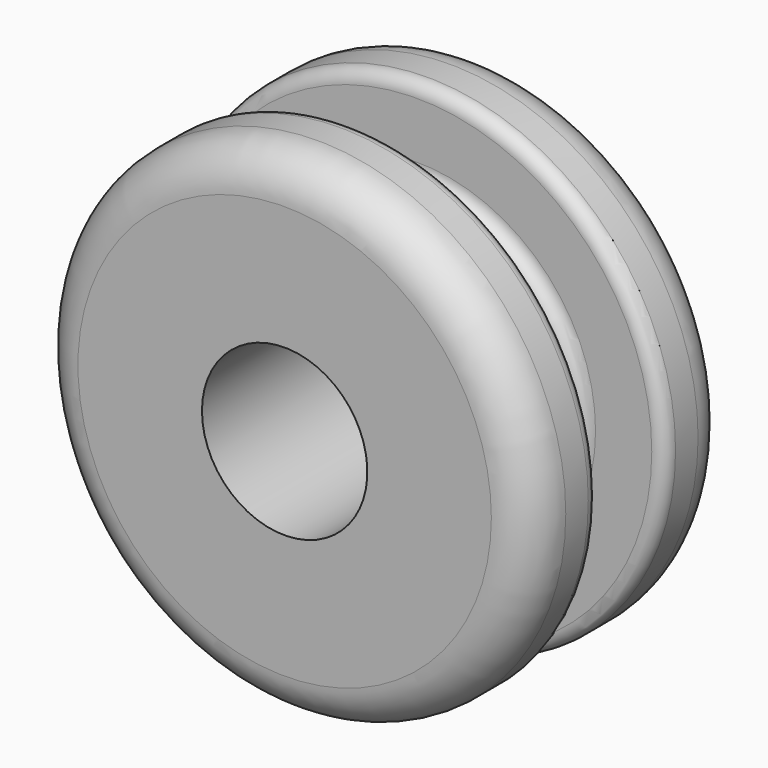
from build123d import *

# Parameters (mm, degrees)
F0_R     = 25.4
F1_DEPTH = 6.35
F2_R     = 38.1
F2_R_2   = 25.4
F3_DEPTH = 12.7
F4_R     = 38.1
F4_R_2   = 25.4
F5_DEPTH = 12.7
F6_R     = 12.7
F7_DEPTH = 38.1
F8_R     = 6.35
F9_R     = 2.032


# Not quite as in the source:
# - a pattern or mirror of a feature is missing from the dataset's text; its kind, count and spacing are read off the source's solid


with BuildPart() as f1:
    # F0 (on Front) → F1 (new body, symmetric)
    with BuildSketch(Plane.XZ):
        Circle(F0_R)
    extrude(amount=F1_DEPTH, both=True)

    # F2 (on face) → F3 (join)
    with BuildSketch(Plane.XZ.offset(6.35)):
        Circle(F2_R)
        Circle(F2_R_2, mode=Mode.SUBTRACT)
        Circle(F2_R_2)
    f3 = extrude(amount=F3_DEPTH)

    # F3_copies: F3 across plane
    add(f3.mirror(Plane.ZX))

    # F4 (on face) → F5 (join)
    with BuildSketch(Plane(origin=(0, 6.35, 0), x_dir=(-1, 0, 0), z_dir=(0, 1, 0))):
        Circle(F4_R)
        Circle(F4_R_2, mode=Mode.SUBTRACT)
    extrude(amount=F5_DEPTH)

    # F6 (on face) → F7 (cut)
    with BuildSketch(Plane(origin=(0, 19.05, 0), x_dir=(-1, 0, 0), z_dir=(0, 1, 0))):
        Circle(F6_R)
    extrude(amount=-F7_DEPTH, mode=Mode.SUBTRACT)

    # F8
    f8_edges = [f1.edges().sort_by_distance(p)[0] for p in [
        (-38.1, 19.05, 0),
        (-38.1, -19.05, 0),
    ]]
    fillet(f8_edges, radius=F8_R)

    # F9
    f9_edges = [f1.edges().sort_by_distance(p)[0] for p in [
        (-25.4, 6.35, 0),
        (-38.1, 6.35, 0),
        (-38.1, -6.35, 0),
        (-25.4, -6.35, 0),
    ]]
    fillet(f9_edges, radius=F9_R)


solid = f1.part
